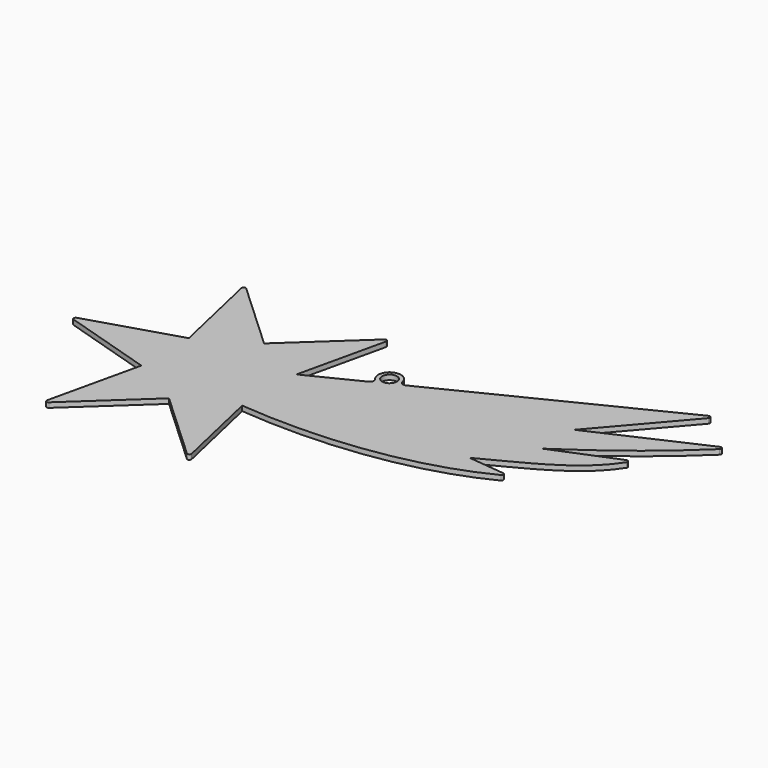
from build123d import *

# Parameters (mm, degrees)
F2_DEPTH = 1
F3_DEPTH = 1
F4_R     = 1.5
F5_DEPTH = 1
F6_R     = 0.8594833568
F7_R     = 0.4


with BuildPart() as f2:
    # F0 (on Top) → F2 (new body)
    with BuildSketch(Plane.XY):
        Polygon((0, 12.0893299047), (-15, 25.9807621135), (-10.4696668122, 6.0446649524), (-30, 0), (-10.4696668122, -6.0446649524), (-15, -25.9807621135), (0, -12.0893299047), (15, -25.9807621135), (10.4696668122, -6.0446649524), (30, 0), (10.4696668122, 6.0446649524), (15, 25.9807621135), align=None)
    extrude(amount=F2_DEPTH)

    # F1 (on Top) → F3 (join)
    with BuildSketch(Plane.XY):
        with BuildLine():
            Line((72.4891722202, 37.6455299556), (7.3894136585, 5.3482959047))
            Line((7.3894136585, 5.3482959047), (7.7781090513, -6.4794942737))
            add(Edge.make_bspline(
                [(58.8173978031, 0.8565816097), (44.8322221637, -6.7676748149), (24.8244935647, -8.4759178571), (7.7781090513, -6.4794942737)],
                knots=[0, 0, 0, 0, 51.5638148865, 51.5638148865, 51.5638148865, 51.5638148865], degree=3))
            add(Edge.make_bspline(
                [(50.0547550619, 1.7504660645), (52.9756359756, 1.4525045796), (55.8965168893, 1.1545430946), (58.8173978031, 0.8565816097)],
                knots=[0, 0, 0, 0, 8.8081176893, 8.8081176893, 8.8081176893, 8.8081176893], degree=3))
            add(Edge.make_bspline(
                [(71.1085945368, 17.1669367701), (66.9464543462, 9.6644256264), (58.5000440478, 6.2858634628), (50.0547550619, 1.7504660645)],
                knots=[0, 0, 0, 0, 26.0946685292, 26.0946685292, 26.0946685292, 26.0946685292], degree=3))
            add(Edge.make_bspline(
                [(57.0727027953, 11.4145213738), (61.7513333758, 13.3319931726), (66.4299639563, 15.2494649713), (71.1085945368, 17.1669367701)],
                knots=[0, 0, 0, 0, 15.1689333795, 15.1689333795, 15.1689333795, 15.1689333795], degree=3))
            add(Edge.make_bspline(
                [(80.8876976371, 30.5125359446), (72.3214372993, 22.1036802977), (66.0250261426, 17.496548593), (57.0727027953, 11.4145213738)],
                knots=[0, 0, 0, 0, 30.5268429396, 30.5268429396, 30.5268429396, 30.5268429396], degree=3))
            add(Edge.make_bspline(
                [(57.0727027953, 19.6979995817), (65.0110344092, 23.302845036), (72.9493660231, 26.9076904903), (80.8876976371, 30.5125359446)],
                knots=[0, 0, 0, 0, 26.155461687, 26.155461687, 26.155461687, 26.155461687], degree=3))
            add(Edge.make_bspline(
                [(72.4891722202, 37.6455299556), (67.3503490786, 31.663019831), (62.2115259369, 25.6805097063), (57.0727027953, 19.6979995817)],
                knots=[0, 0, 0, 0, 23.6596994075, 23.6596994075, 23.6596994075, 23.6596994075], degree=3))
        make_face()
    extrude(amount=F3_DEPTH)

    # F4 (on face) → F5 (join)
    with BuildSketch(Plane(origin=(0, 0, 0), x_dir=(1, 0, 0), z_dir=(0, 0, -1))):
        with BuildLine():
            ThreePointArc((22.4657231152, -12.8279410816), (21.8424371227, -16.8758669464), (25.489, -15.011257492))
            ThreePointArc((25.489, -15.011257492), (25.4577954947, -14.6336770325), (25.3650286927, -14.2663419742))
            Line((25.3650286927, -14.2663419742), (22.4657231152, -12.8279410816))
        make_face()
        with Locations((23.189, -15.011257492)):
            Circle(F4_R, mode=Mode.SUBTRACT)
    extrude(amount=-F5_DEPTH)

    # F6
    f6_edges = [f2.edges().sort_by_distance(p)[0] for p in [
        (25.489, 15.011257, 0.5),
        (25.365029, 14.266342, 0.5),
        (22.465723, 12.827941, 0.5),
    ]]
    fillet(f6_edges, radius=F6_R)

    # F7
    f7_edges = [f2.edges().sort_by_distance(p)[0] for p in [
        (15, 25.980762, 0.5),
        (-15, 25.980762, 0.5),
        (-30, 0, 0.5),
        (-15, -25.980762, 0.5),
        (15, -25.980762, 0.5),
        (72.489172, 37.64553, 0.5),
        (80.887698, 30.512536, 0.5),
        (71.108595, 17.166937, 0.5),
        (58.817398, 0.856582, 0.5),
    ]]
    fillet(f7_edges, radius=F7_R)


solid = f2.part
